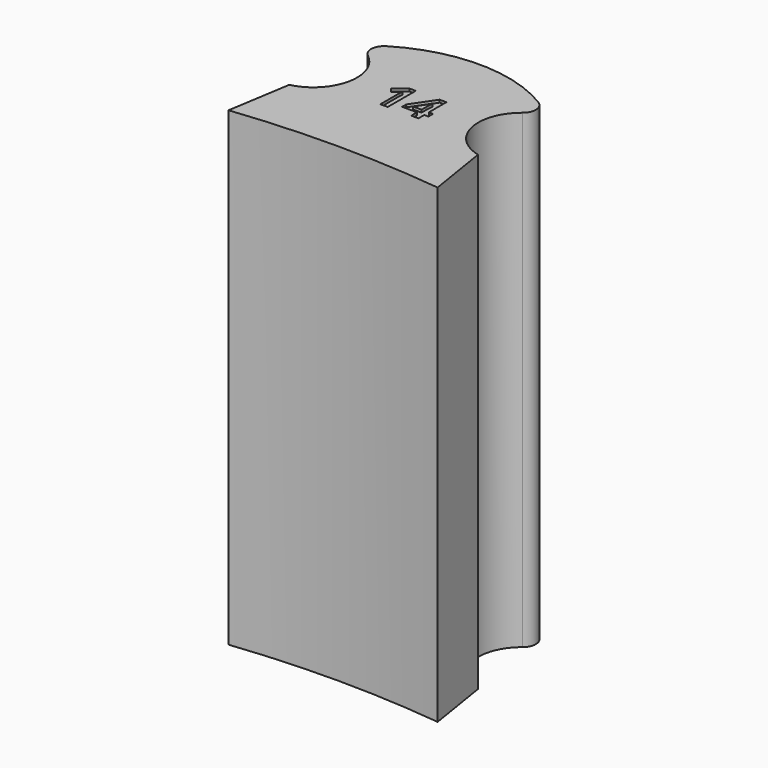
from build123d import *

# Parameters (mm, degrees)
F1_DEPTH     = 180
F2_TEXT_SIZE = 18.7331137972
F3_DEPTH     = 1


# Not quite as in the source:
# - Text() gives the source's letters only with a copy of the font that has no kerning and outlines rounded to 1/6400 em; it was checked with that copy


with BuildPart() as f1:
    # F0 (on Top) → F1 (new body)
    with BuildSketch(Plane.XY):
        with BuildLine():
            Line((3.8687128108, 24.1569802165), (0, 0))
            ThreePointArc((0, 0), (40, 2.2607195109), (80, 0))
            Line((80, 0), (76.1312871892, 24.1569802165))
            ThreePointArc((76.1312871892, 24.1569802165), (63.5975554576, 36.8458138953), (69.5972800683, 53.6417728094))
            ThreePointArc((69.5972800683, 53.6417728094), (71.4969098635, 57.8715436357), (69.1043731597, 61.843359684))
            ThreePointArc((69.1043731597, 61.843359684), (40, 70), (10.8956268403, 61.843359684))
            ThreePointArc((10.8956268403, 61.843359684), (8.5030901365, 57.8715436357), (10.4027199317, 53.6417728094))
            ThreePointArc((10.4027199317, 53.6417728094), (16.4024445424, 36.8458138953), (3.8687128108, 24.1569802165))
        make_face()
    extrude(amount=F1_DEPTH)

    # F2 (on face) → F3 (cut)
    with BuildSketch(Plane.XY.offset(180)):
        with Locations((28.077268973, 31.3721522689)):
            Text('14', F2_TEXT_SIZE, font='Open Sans', font_style=FontStyle.BOLD, text_align=(TextAlign.LEFT, TextAlign.BOTTOM))
    extrude(amount=-F3_DEPTH, mode=Mode.SUBTRACT)


solid = f1.part
